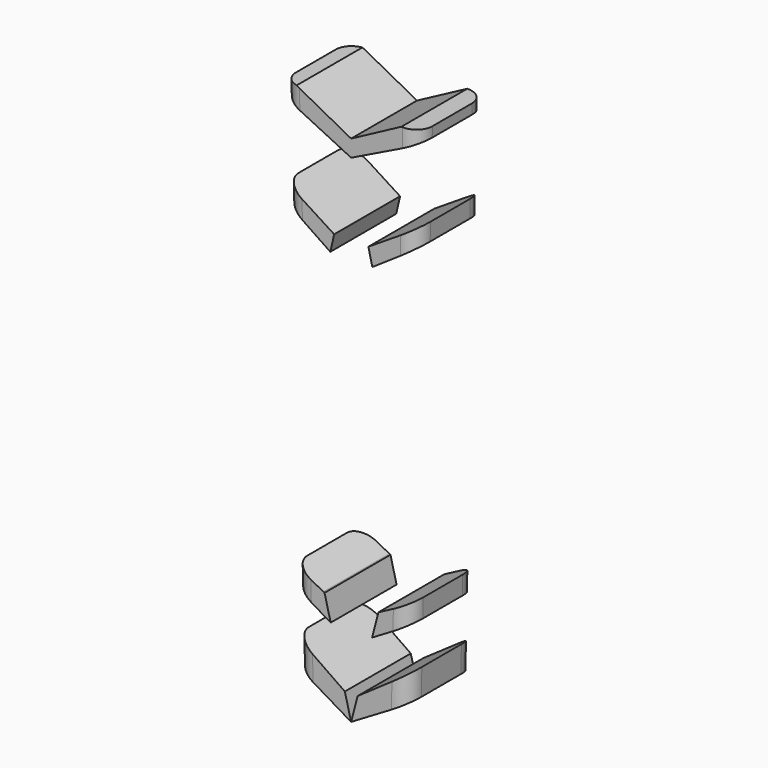
from build123d import *

# Parameters (mm, degrees)
F1_DEPTH = 6.35
F2_DEPTH = 6.35
F4_DEPTH = 25.4
F5_R     = 2.54


with BuildPart() as f1:
    # F0 (on Front) → F1 (new body)
    with BuildSketch(Plane.XZ):
        Polygon((10.5009634349, -8.6313571018), (0, -8.4001217037), (-10.5245159939, -8.168367669), (-8.3013391122, -91.856867075), (8.6683045514, -91.856867075), align=None)
    extrude(amount=F1_DEPTH)

    # F2 (add): a face of the model
    f2_faces = [f1.faces().sort_by_distance(p)[0] for p in [
        (0.0745348421, 0, -48.6438367355),
    ]]
    extrude(f2_faces, amount=F2_DEPTH)

    # F3 (on face) → F4 (cut)
    with BuildSketch(Plane.XZ.offset(6.35)):
        Polygon((-8.4089043082, -8.2149542811), (0, -12.6956291497), (7.741477061, -8.5705921125), align=None)
        Polygon((0, -15.2933746576), (-10.4707083295, -10.1938847244), (-10.1647846318, -21.7099702861), (-2.6734457948, -26.4930181658), (-2.660532576, -26.5012629595), (-2.6115273083, -26.532551698), align=None)
        Polygon((10.2136542458, -21.6787681594), (10.4665109394, -10.1959289555), (0, -15.2933746576), (2.660532576, -26.5012629595), align=None)
        Polygon((2.660532576, -26.5012629595), (0, -15.2933746576), (-2.6115273083, -26.532551698), (-3.2102312503, -29.1091816943), (-9.2748739024, -55.2094611118), (-4.0967862529, -75.6694136894), (-3.1505538377, -79.4082206875), (-0.965611629, -88.0414878319), (0, -91.856867075), (0.9910429813, -88.023830283), (3.2309755221, -79.3604887305), (4.199302435, -75.6153104147), (9.4752950296, -55.2094611118), (3.2699760565, -29.068634063), align=None)
        Polygon((-3.4606218927, -28.9392464633), (-10.0923027152, -24.4384544155), (-9.2748739024, -55.2094611118), (-3.2102312503, -29.1091816943), (-3.2699760565, -29.068634063), align=None)
        Polygon((9.4752950296, -55.2094611118), (10.15380398, -24.3967147102), (3.2699760565, -29.068634063), align=None)
        Polygon((-4.0967862529, -75.6694136894), (-9.2748739024, -55.2094611118), (-8.7972565245, -73.1887240187), (-4.2695118804, -75.5782571337), (-4.199302435, -75.6153104147), align=None)
        Polygon((9.0827017549, -73.0380792973), (9.4752950296, -55.2094611118), (4.199302435, -75.6153104147), align=None)
        Polygon((-0.965611629, -88.0414878319), (-3.1505538377, -79.4082206875), (-3.2309755221, -79.3604887305), (-3.3105833326, -79.3132398248), (-8.7198462703, -76.1027287805), (-8.5424459568, -82.7807246478), (-1.0061214638, -88.0133609601), (-0.9910429813, -88.023830283), align=None)
        Polygon((9.0191284413, -75.9250985328), (3.2309755221, -79.3604887305), (0.9910429813, -88.023830283), (8.8732221424, -82.5510594467), align=None)
        Polygon((-8.3013391122, -91.856867075), (0, -91.856867075), (-8.434321605, -86.8509202434), align=None)
        Polygon((8.7830958233, -86.6439154273), (0, -91.856867075), (8.6683045514, -91.856867075), align=None)
    extrude(amount=-F4_DEPTH, mode=Mode.SUBTRACT)

    # F5
    f5_edges = [f1.edges().sort_by_distance(p)[0] for p in [
        (-10.497612, -6.35, -9.181126),
        (-10.128544, -6.35, -23.074212),
        (-8.758551, -6.35, -74.645726),
        (-8.488384, -6.35, -84.815822),
        (-8.758551, 6.35, -74.645726),
        (-8.488384, 6.35, -84.815822),
        (9.050915, -6.35, -74.481589),
        (8.828159, -6.35, -84.597487),
        (-10.497612, 6.35, -9.181126),
        (-10.128544, 6.35, -23.074212),
        (10.183729, -6.35, -23.037741),
        (10.483737, -6.35, -9.413643),
        (10.483737, 6.35, -9.413643),
        (10.183729, 6.35, -23.037741),
        (8.828159, 6.35, -84.597487),
        (9.050915, 6.35, -74.481589),
    ]]
    fillet(f5_edges, radius=F5_R)


solid = f1.part
